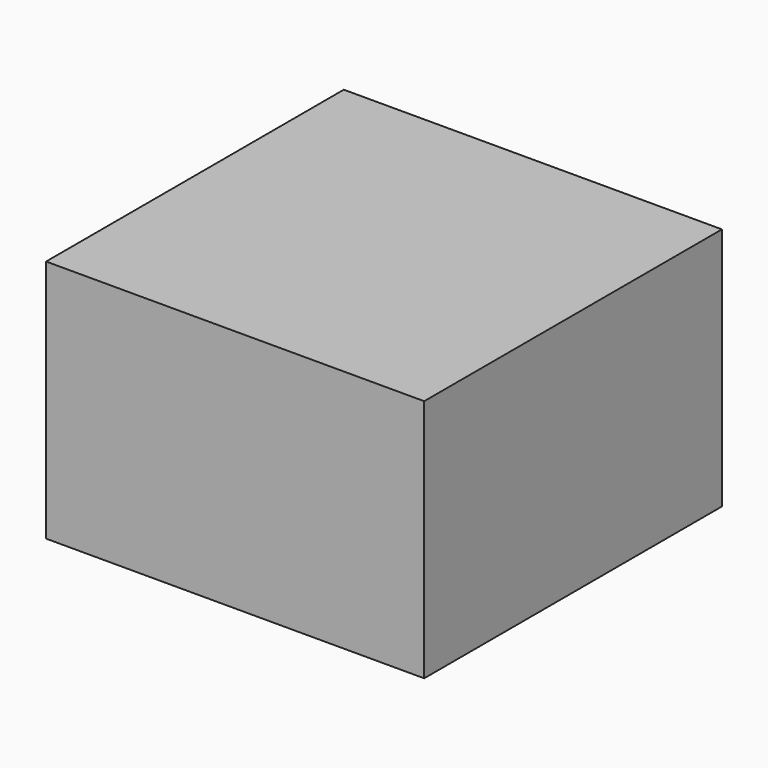
from build123d import *

# Parameters (mm, degrees)
F0_W     = 69.8630958796
F0_H     = 137.5265717506
F2_DEPTH = 90.1570245624


# Not quite as in the source:
# - the program builds the solid bodies; features that only make, move or delete a surface that nothing else refers to are left out


with BuildPart() as f2:
    # F0 (on Top) → F2 (new body)
    with BuildSketch(Plane.XY):
        with Locations((-34.9315479398, 0)):
            Rectangle(F0_W, F0_H)
        with Locations((34.9315479398, 0)):
            Rectangle(F0_W, F0_H)
    extrude(amount=-F2_DEPTH)


solid = f2.part
